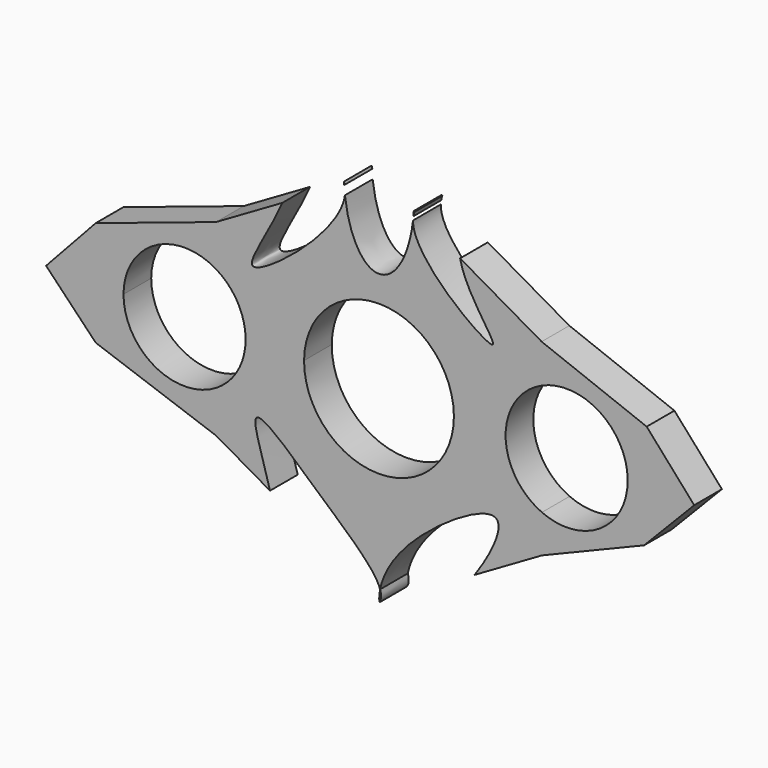
from build123d import *

# Parameters (mm, degrees)
F1_DEPTH = 5.08


with BuildPart() as f1:
    # F0 (on Front) → F1 (new body)
    with BuildSketch(Plane.XZ):
        with BuildLine():
            Line((23.8544226128, 13.8363139495), (11.8995172721, 20.7065034498))
            add(Edge.make_bspline(
                [(11.8995172721, 20.7065034498), (12.7527047238, 16.3214990301), (23.6984449015, 4.8622046649), (4.8911049153, 18.4580126576), (4.9955159434, 23.3538565741)],
                knots=[0, 0, 0, 0, 0.2510815361, 0.566393336, 0.566393336, 0.566393336, 0.566393336], degree=3))
            add(Edge.make_bspline(
                [(-4.9955159434, 23.3538565741), (-4.0065950779, 14.8329585791), (0, 14.8329585791), (4.0065950779, 14.8329585791), (4.9955159434, 23.3538565741)],
                knots=[1.8201970434, 1.8201970434, 1.8201970434, 3.1415926536, 3.1415926536, 4.4629882638, 4.4629882638, 4.4629882638], degree=2, weights=[1, 0.7895642031, 1, 0.7895642031, 1]))
            add(Edge.make_bspline(
                [(-14.1796024948, 19.3842051979), (-16.1087852311, 14.8596253569), (-24.5159632533, 3.3211353455), (-5.6744217692, 18.0019188802), (-4.9955159434, 23.3538565741)],
                knots=[0, 0, 0, 0, 0.2419326445, 0.5682555357, 0.5682555357, 0.5682555357, 0.5682555357], degree=3))
            Line((-14.1796024948, 19.3842051979), (-23.9098106814, 13.7403790006))
            Line((-23.9098106814, 13.7403790006), (-23.8976251995, 7.6734533511))
            ThreePointArc((-23.8976251995, 7.6734533511), (-20.730112215, 4.4297703221), (-19.5576464714, 0.0502792352))
            Line((-19.5576464714, 0.0502792352), (-10.9852926415, 0.0674968952))
            ThreePointArc((-10.9852926415, 0.0674968952), (-0.0220644441, 10.9854778417), (10.9849328747, 0.1116243169))
            Line((10.9849328747, 0.1116243169), (18.5708946822, 0.1268607984))
            ThreePointArc((18.5708946822, 0.1268607984), (20.0443809343, 4.922194791), (23.8657988515, 8.1722955491))
            Line((23.8657988515, 8.1722955491), (23.8544226128, 13.8363139495))
        make_face()
        with BuildLine():
            Line((39.2630137504, 7.8735761344), (23.8544226128, 13.8363139495))
            Line((23.8544226128, 13.8363139495), (23.8657988515, 8.1722955491))
            ThreePointArc((23.8657988515, 8.1722955491), (32.3240559978, 7.557763228), (36.4755152887, 0.1628224112))
            Line((36.4755152887, 0.1628224112), (41.5712800692, 0.1730573066))
            Line((41.5712800692, 0.1730573066), (41.5622201778, 4.6838093397))
            Line((41.5622201778, 4.6838093397), (39.2630137504, 7.8735761344))
        make_face()
        Polygon((46.2305024266, 0), (39.2630137504, 7.8735761344), (41.5622201778, 4.6838093397), (41.5712800692, 0.1730573066), (41.5716276565, 0), (38.8891281875, -7.569654379), align=None)
        with BuildLine():
            Line((41.5712800692, 0.1730573066), (36.4755152887, 0.1628224112))
            ThreePointArc((36.4755152887, 0.1628224112), (36.4766257405, 0.0814145715), (36.4769959013, 0))
            ThreePointArc((36.4769959013, 0), (32.4076622958, -7.504004323), (23.8986565077, -8.1869225977))
            Line((23.8986565077, -8.1869225977), (23.9098106814, -13.7403790006))
            Line((23.9098106814, -13.7403790006), (38.8891281875, -7.569654379))
            Line((38.8891281875, -7.569654379), (41.5716276565, 0))
            Line((41.5716276565, 0), (41.5712800692, 0.1730573066))
        make_face()
        with BuildLine():
            ThreePointArc((23.8986565077, -8.1869225977), (19.9850775207, -4.830880931), (18.5708946822, 0.1268607984))
            Line((18.5708946822, 0.1268607984), (10.9849328747, 0.1116243169))
            ThreePointArc((10.9849328747, 0.1116243169), (10.9853582178, 0.0558128788), (10.9855, 0))
            ThreePointArc((10.9855, 0), (-0.0337486069, -10.9854481602), (-10.9852926415, 0.0674968952))
            Line((-10.9852926415, 0.0674968952), (-19.5576464714, 0.0502792352))
            ThreePointArc((-19.5576464714, 0.0502792352), (-19.5575405901, 0.0251397167), (-19.5575052963, 0))
            ThreePointArc((-19.5575052963, 0), (-20.7088673521, -4.3922438172), (-23.8668381271, -7.6548594732))
            Line((-23.8668381271, -7.6548594732), (-23.8544226128, -13.8363139495))
            Line((-23.8544226128, -13.8363139495), (-15.9790920253, -18.3620723701))
            add(Edge.make_bspline(
                [(0.163388369, -25.8532824823), (-0.5824883081, -23.5445287745), (-8.8142073886, -16.5809605771), (-20.7736627649, -5.1912645148), (-16.9995624931, -14.3564310957), (-15.9790920253, -18.3620723701)],
                knots=[0.0461674631, 0.0461674631, 0.0461674631, 0.0461674631, 0.2131983653, 0.4232173263, 0.6005724186, 0.6005724186, 0.6005724186, 0.6005724186], degree=3))
            add(Edge.make_bspline(
                [(0.163388369, -25.8532824823), (0.5984234349, -23.6166229337), (4.4335734026, -16.9603900208), (20.3472971341, -7.0641553228), (16.8185248338, -15.4600803358), (14.0872810007, -19.3800999399), (14.0188094193, -19.4774702293)],
                knots=[0.0441354144, 0.0441354144, 0.0441354144, 0.0441354144, 0.2056976035, 0.4443926766, 0.6304870786, 0.6352232986, 0.6352232986, 0.6352232986, 0.6352232986], degree=3))
            Line((14.0188094193, -19.4774702293), (23.9098106814, -13.7403790006))
            Line((23.9098106814, -13.7403790006), (23.8986565077, -8.1869225977))
        make_face()
        with BuildLine():
            Line((-23.8976251995, 7.6734533511), (-23.9098106814, 13.7403790006))
            Line((-23.9098106814, 13.7403790006), (-41.5380969644, 7.8735761344))
            Line((-41.5380969644, 7.8735761344), (-44.5907459629, 4.5725049953))
            Line((-44.5907459629, 4.5725049953), (-44.5907459629, 0))
            Line((-44.5907459629, 0), (-37.4644938557, 0.0143131499))
            ThreePointArc((-37.4644938557, 0.0143131499), (-32.9126802641, 7.7968211297), (-23.8976251995, 7.6734533511))
        make_face()
        with BuildLine():
            ThreePointArc((-23.8668381271, -7.6548594732), (-32.9094839983, -7.7986247094), (-37.4644938557, 0.0143131499))
            Line((-37.4644938557, 0.0143131499), (-44.5907459629, 0))
            Line((-44.5907459629, 0), (-44.5907459629, -2.3883581161))
            Line((-44.5907459629, -2.3883581161), (-41.5380969644, -7.569654379))
            Line((-41.5380969644, -7.569654379), (-23.8544226128, -13.8363139495))
            Line((-23.8544226128, -13.8363139495), (-23.8668381271, -7.6548594732))
        make_face()
        Polygon((-44.5907459629, 0), (-44.5907459629, 4.5725049953), (-48.8191470504, 0), (-41.5380969644, -7.569654379), (-44.5907459629, -2.3883581161), align=None)
    extrude(amount=F1_DEPTH)


with BuildPart() as f1b:
    # F0 (on Front) → F1, piece 2 (new body)
    with BuildSketch(Plane.XZ):
        with BuildLine():
            add(Edge.make_bspline(
                [(5.05297105, 23.9064308163), (5.0935955947, 24.1228884346), (5.1546696758, 24.333291686), (5.2336305106, 24.5372243074)],
                knots=[0.5785155836, 0.5785155836, 0.5785155836, 0.5785155836, 0.5930865518, 0.5930865518, 0.5930865518, 0.5930865518], degree=3))
            Line((5.2336305106, 24.5372243074), (5.1072520142, 24.609850915))
            add(Edge.make_bspline(
                [(5.05297105, 23.9064308163), (5.085167197, 24.2562618556), (5.1072520142, 24.609850915)],
                knots=[4.5130919957, 4.5130919957, 4.5130919957, 4.5761642718, 4.5761642718, 4.5761642718], degree=2, weights=[1, 0.9995027772, 1]))
        make_face()
    extrude(amount=F1_DEPTH)


with BuildPart() as f1c:
    # F0 (on Front) → F1, piece 3 (new body)
    with BuildSketch(Plane.XZ):
        with BuildLine():
            add(Edge.make_bspline(
                [(-5.1321122684, 25.0811244519), (-5.1226991178, 24.8626735882), (-5.1094332892, 24.6451880664)],
                knots=[1.6650830677, 1.6650830677, 1.6650830677, 1.7038689923, 1.7038689923, 1.7038689923], degree=2, weights=[1, 0.9998119624, 1]))
            Line((-5.1094332892, 24.6451880664), (-5.0355162164, 24.688062289))
            add(Edge.make_bspline(
                [(-5.0355162164, 24.688062289), (-5.0614762451, 24.822005601), (-5.0938469313, 24.9530733475), (-5.1321122684, 25.0811244519)],
                knots=[0.596906543, 0.596906543, 0.596906543, 0.596906543, 0.6060843122, 0.6060843122, 0.6060843122, 0.6060843122], degree=3))
        make_face()
    extrude(amount=F1_DEPTH)


with BuildPart() as f1d:
    # F0 (on Front) → F1, piece 4 (new body)
    with BuildSketch(Plane.XZ):
        with BuildLine():
            add(Edge.make_bspline(
                [(0.0553880686, -27.5766929501), (0.0087635928, -27.0417101596), (0.0445458786, -26.464291138), (0.163388369, -25.8532824823)],
                knots=[0, 0, 0, 0, 0.0441354144, 0.0441354144, 0.0441354144, 0.0441354144], degree=3))
            add(Edge.make_bspline(
                [(0.0553880686, -27.5766929501), (0.3541021804, -27.0702754536), (0.3695492259, -26.4914236891), (0.163388369, -25.8532824823)],
                knots=[0, 0, 0, 0, 0.0461674631, 0.0461674631, 0.0461674631, 0.0461674631], degree=3))
        make_face()
    extrude(amount=F1_DEPTH)


solid = Compound([f1.part, f1b.part, f1c.part, f1d.part])
